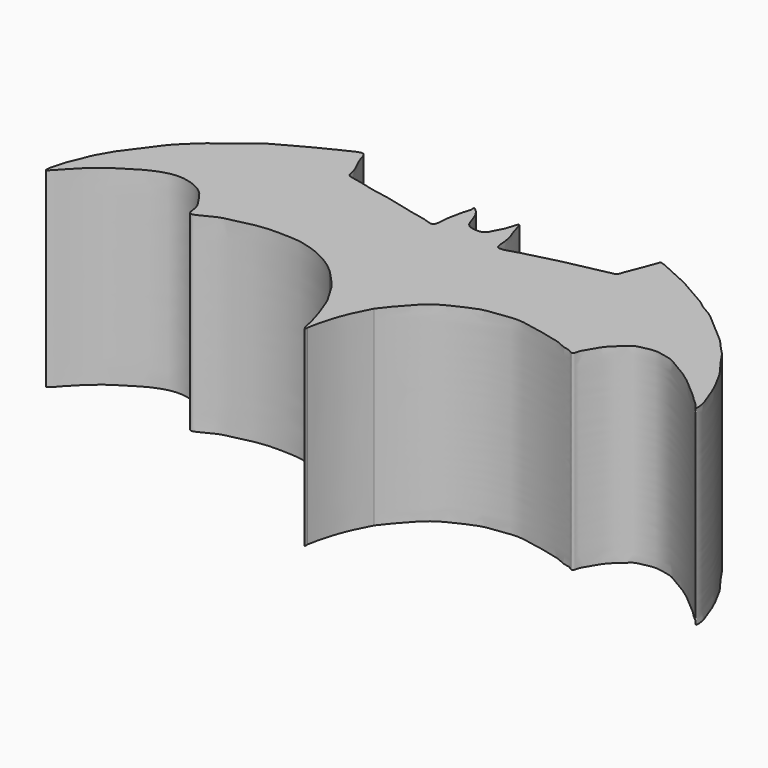
from build123d import *

# Parameters (mm, degrees)
F1_DEPTH = 25


# Not quite as in the source:
# - ends of sketch curves that miss each other by under 0.0002 mm in the source are joined


with BuildPart() as f1:
    # F0 (on Top) → F1 (new body)
    with BuildSketch(Plane.XY):
        with BuildLine():
            add(Edge.make_bspline(
                [(-40.1968471706, -23.0873599648), (-40.0821652579, -22.6443739225), (-39.8639632828, -21.8015171271), (-39.5435051275, -20.7789783314), (-38.9624616028, -19.5766025839), (-38.6248192553, -18.4622828305), (-37.8764356227, -17.1896178035), (-37.3223083399, -16.1426343346), (-36.5033448154, -15.1406645327), (-35.5671807336, -13.8474938719), (-34.7404028099, -12.6619867692), (-33.7213474012, -11.3367760015), (-32.5709136851, -10.2726462551), (-31.2488039384, -8.9161188537), (-29.477712685, -7.7490635161), (-27.9115017025, -6.3352311912), (-26.4610965168, -5.1672752357), (-24.8469714717, -4.3815980141), (-22.76616761, -3.1267258394), (-20.197558566, -1.922936453), (-18.4645703482, -0.9889353135), (-16.9432166525, -0.3776336266), (-16.7241377526, -1.7472285966), (-16.0983957866, -2.98061749), (-15.3865504555, -4.3875457176), (-15.4694646208, -5.5339323373), (-13.5571991944, -5.6849648844), (-12.1076010518, -6.2221198071), (-9.8030724141, -6.5819033007), (-7.8777646095, -6.9888346023), (-5.5731675689, -7.6921919678), (-3.3170197485, -7.9683608609), (-1.5592142712, -8.8156744244), (-1.5875609412, -7.0755561172), (-1.3908853453, -5.9424344394), (-1.0948496289, -4.3876609047), (-0.696817184, -3.4472296341), (-0.9233984107, -2.7627548299), (0.2207261996, -3.7487128755), (0.6575865872, -5.0913132804), (1.05768838, -6.3661599967), (2.0957548088, -6.7557202463), (3.5664498521, -6.7239926634), (3.9815612421, -5.4706314467), (4.6509078444, -4.5968960366), (5.105251181, -2.2333464779), (5.5436434557, -4.3830876586), (5.9072053976, -5.0882691082), (6.4130563138, -6.8514311697), (6.3013952004, -8.8147866429), (8.7884804661, -7.8344097925), (10.6362955306, -7.500438229), (13.2736835098, -6.718549896), (15.4951850723, -6.2631292249), (18.0080425407, -5.7448091068), (19.1432502742, -5.5047284656), (19.6511745453, -5.3973095492)],
                knots=[0, 0, 0, 0, 0.0170610068, 0.0324614868, 0.0493612671, 0.0655218559, 0.0833760304, 0.0995162111, 0.1162878049, 0.1349643643, 0.1529261659, 0.1719058297, 0.1904741087, 0.2107547548, 0.2324081495, 0.253991647, 0.2740258308, 0.2936779511, 0.3168600822, 0.3419419356, 0.3634207404, 0.3798087119, 0.3948608713, 0.4129569613, 0.4315237718, 0.4455150974, 0.4642344254, 0.4834313288, 0.5057165451, 0.526728373, 0.549601706, 0.5727777848, 0.5902520588, 0.606636694, 0.6234810643, 0.6420748776, 0.6573039245, 0.6659640514, 0.6810636629, 0.6998007085, 0.7161858288, 0.7312401883, 0.748088179, 0.7637244879, 0.7808563694, 0.7987563178, 0.8154519605, 0.8302664091, 0.8503849202, 0.8679699115, 0.8888959441, 0.9104372868, 0.9345698574, 0.9573471235, 0.9809158883, 1, 1, 1, 1], degree=3))
            add(Edge.make_bspline(
                [(-3.6454189103, -23.0655353516), (-3.9700357905, -22.7804086809), (-4.688111127, -22.1496884611), (-6.3989491613, -21.0839150655), (-8.2799567849, -20.3231216792), (-10.1946000306, -19.8356650727), (-12.1145921887, -19.7683859316), (-14.0816405812, -19.7235863275), (-16.1779945431, -19.9789483234), (-18.1918308983, -20.5578474853), (-20.1207526826, -20.7918932665), (-23.0313163117, -22.8266895653), (-22.9045006793, -20.5727904096), (-23.8014948384, -19.4081332415), (-24.7427870508, -17.8290780293), (-26.234027042, -16.8692420735), (-28.1800156141, -16.3098850154), (-30.0253338558, -16.466795709), (-32.0381815128, -17.2364274948), (-33.6649628124, -18.2571987271), (-35.7691363818, -19.5433076538), (-37.192892414, -20.7539734971), (-38.6406714979, -22.2063984812), (-39.2698386612, -22.9741411763), (-40.3722264802, -24.143950946), (-40.2509312224, -23.4131949876), (-40.1968471706, -23.0873599648)],
                knots=[0, 0, 0, 0, 0.0363086698, 0.0803173275, 0.1249387314, 0.1684429741, 0.2113865674, 0.2550125042, 0.3002441538, 0.3444521462, 0.3903745582, 0.440702162, 0.4770983378, 0.515879267, 0.5574217063, 0.5985220635, 0.6422084742, 0.684408794, 0.7294324381, 0.773070489, 0.8214485683, 0.864952819, 0.9083589752, 0.9422417588, 0.9742463163, 1, 1, 1, 1], degree=3))
            add(Edge.make_bspline(
                [(0.5723864888, -29.0262363851), (0.4682378359, -28.7586663924), (0.2822454991, -28.280830464), (-0.0116444167, -27.8905766618), (-0.3677904467, -27.1838078721), (-0.7717775214, -26.5846935372), (-1.3210933045, -25.5412114338), (-2.3684793038, -24.4038900115), (-3.2068699188, -23.5251765777), (-3.6454189103, -23.0655353516)],
                knots=[0, 0, 0, 0, 0.1273527951, 0.2274311123, 0.3516788503, 0.4740505874, 0.6265403472, 0.8046491085, 1, 1, 1, 1], degree=3))
            add(Edge.make_bspline(
                [(2.4690291857, -34.3355481578), (2.4868411073, -34.5368452574), (2.52720507, -34.9930087618), (2.0401125993, -34.0909924777), (2.0463543441, -33.3579315615), (1.7799086579, -32.5211803088), (1.567968678, -31.6672622635), (1.1890119666, -30.7043768415), (0.9028633326, -29.7954955647), (0.6798280471, -29.2763307762), (0.5723864888, -29.0262363851)],
                knots=[0, 0, 0, 0, 0.0895468266, 0.2029239087, 0.331009591, 0.4598799076, 0.592166599, 0.7349606271, 0.8723240442, 1, 1, 1, 1], degree=3))
            add(Edge.make_bspline(
                [(5.1556448452, -26.7993882298), (5.0353945307, -27.0134990148), (4.7914675536, -27.4478213431), (4.4725552741, -28.1596144069), (4.1025298063, -28.823997989), (3.9009480623, -29.4322693079), (3.6809253051, -29.9391885154), (3.4493076689, -30.5257635178), (3.2068145088, -31.3026010991), (3.0224463474, -31.9056179295), (2.8719974676, -32.522433859), (2.7218207152, -33.061841374), (2.6431061637, -33.4685907164), (2.5144634178, -34.1083247268), (2.4780655945, -34.2903228506), (2.4690291857, -34.3355481578)],
                knots=[0, 0, 0, 0, 0.0846948955, 0.1718030421, 0.2577687976, 0.3361122532, 0.4084807072, 0.486824265, 0.5755572637, 0.6543262562, 0.7327200822, 0.8050887195, 0.8704953712, 0.9525978604, 0.9845372386, 0.9845372386, 0.9845372386, 0.9845372386], degree=3))
            add(Edge.make_bspline(
                [(30.4335709661, -4.8713628203), (30.7107146067, -5.1150183022), (31.284034491, -5.6190620984), (32.4641591981, -6.133565822), (33.6650360911, -7.1498779185), (34.8336375284, -8.1852374152), (35.8542930312, -9.1117153158), (37.1131496437, -10.0037353672), (38.1171132809, -11.344242795), (39.3497914289, -12.4364125598), (40.2453545191, -14.0438105296), (41.7565501877, -15.8276788154), (42.5613405142, -17.4477672213), (43.4688048285, -19.0915626473), (43.9990375547, -20.8073713207), (44.6557284, -22.1525183208), (44.7154224009, -23.8306131029), (44.0920911693, -22.7129185747), (43.3066654105, -22.199651566), (42.6198743859, -21.3610579976), (41.3709144463, -20.4538875113), (40.6003837602, -19.6606375305), (39.5311411521, -18.8161944963), (38.3149121196, -17.9945420755), (36.9624715916, -17.2775877098), (35.9313452806, -16.5440446386), (34.478689866, -16.2929132669), (33.4545560154, -16.0598035569), (32.1596741001, -16.3564652317), (30.9073852743, -16.5970708586), (30.4572399618, -17.2149150379), (29.6012949555, -17.8833968703), (28.6876304241, -18.7849216976), (27.9452867803, -20.2497254903), (27.3851896879, -20.9994607354), (27.2657563672, -22.0983396605), (26.5050215865, -21.4129035781), (25.6863266722, -21.4167237107), (24.7326719559, -20.8711149716), (23.837225, -20.6357916093), (22.6414772635, -20.3717949694), (21.4901935981, -20.0573315634), (20.2167346659, -19.9188557401), (18.9172982176, -19.5207541036), (17.2482501029, -19.5773916779), (15.4739299687, -19.8077644565), (13.9176711013, -20.0263342828), (12.4787419381, -20.6418192455), (10.6573964904, -21.4536764033), (9.026320295, -22.3809902828), (7.4377623347, -23.9810269902), (5.8617231519, -25.8575340842), (5.3590928518, -26.5280042394), (5.1556448452, -26.7993882298)],
                knots=[0, 0, 0, 0, 0.0176467809, 0.0365054394, 0.0575240525, 0.0784817826, 0.0980917649, 0.1187473953, 0.1403477195, 0.1616145338, 0.1843270232, 0.2098409107, 0.2324647985, 0.2552648794, 0.2775489539, 0.2992693062, 0.3163163351, 0.3306670087, 0.347637782, 0.3649980864, 0.3856537168, 0.4034125698, 0.4227037934, 0.4431760026, 0.4637996093, 0.4826582678, 0.5026431159, 0.5197654106, 0.539069676, 0.5575979936, 0.571752053, 0.58888744, 0.6081261706, 0.6293832251, 0.646296093, 0.660741095, 0.6745543541, 0.6900345426, 0.7072126418, 0.7234455447, 0.7418396318, 0.7602337189, 0.7790361593, 0.798431101, 0.819994091, 0.8425118866, 0.8633254161, 0.8841907829, 0.9077443523, 0.9305839137, 0.9559611161, 0.9821745264, 1, 1, 1, 1], degree=3))
            add(Edge.make_bspline(
                [(21.646939218, -0.4653866636), (21.8579533435, -0.5211374089), (22.3031494521, -0.6387599369), (23.0100796409, -1.04718797), (23.9640461844, -1.4162903333), (24.7554440955, -1.8147290906), (25.6832878281, -2.2149391819), (26.6371658613, -2.6391001705), (27.5699629481, -3.2315523697), (28.3822846288, -3.6394607094), (29.928174179, -4.6266741672), (30.3013671526, -4.8073561351), (30.4335709661, -4.8713628203)],
                knots=[0, 0, 0, 0, 0.0830542194, 0.1752272044, 0.2782447684, 0.3747029573, 0.4765435803, 0.5817564955, 0.6865050602, 0.787766681, 0.9248162316, 1, 1, 1, 1], degree=3))
            add(Edge.make_bspline(
                [(19.6511745453, -5.3973095492), (19.7326220313, -5.3381285215), (19.9227341418, -5.1999900642), (20.0402859922, -4.6044381365), (20.2636083703, -4.1389711306), (20.7265788768, -2.9663823761), (21.0592352836, -2.0660907768), (21.3816918606, -1.1023058118), (21.5642265667, -0.663998525), (21.646939218, -0.4653866636)],
                knots=[0, 0, 0, 0, 0.09366565, 0.2186313573, 0.3419052005, 0.5268160582, 0.6958417099, 0.8621755878, 1, 1, 1, 1], degree=3))
        make_face()
    extrude(amount=F1_DEPTH)


solid = f1.part
